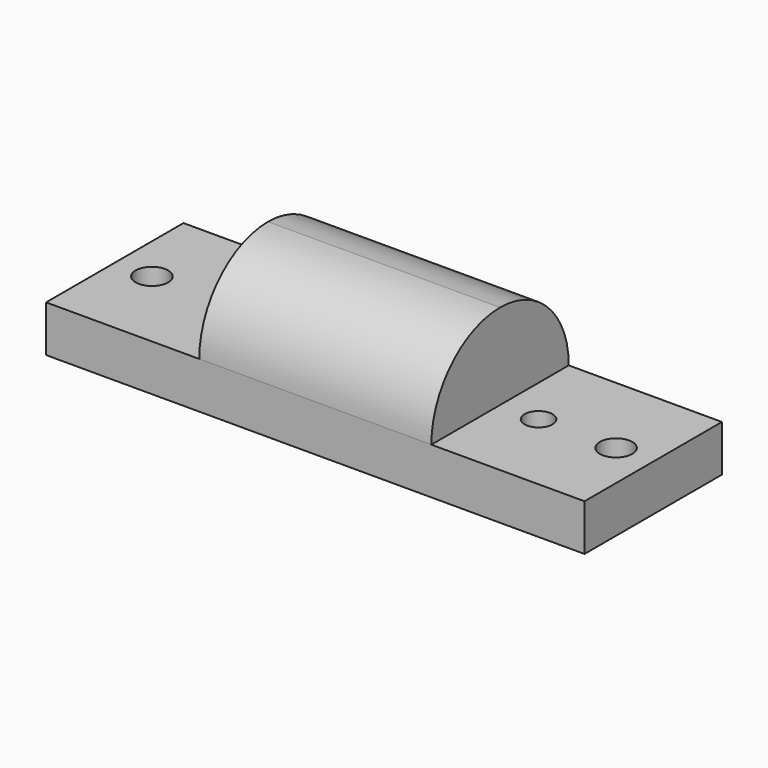
from build123d import *

# Parameters (mm, degrees)
F0_W     = 38
F0_H     = 18.5
F0_R     = 1.5
F0_W_2   = 10
F0_R_2   = 1.75
F1_DEPTH = 5
F2_W     = 25
F2_H     = 18.5
F3_DEPTH = 9.25
F5_DEPTH = 25


with BuildPart() as f1:
    # F0 (on Top) → F1 (new body)
    with BuildSketch(Plane.XY):
        Rectangle(F0_W, F0_H)
        with Locations((-16.65, 0)):
            Circle(F0_R, mode=Mode.SUBTRACT)
        with Locations((16.65, 0)):
            Circle(F0_R, mode=Mode.SUBTRACT)
        with Locations((24, 0)):
            Rectangle(F0_W_2, F0_H)
        with Locations((25, 0)):
            Circle(F0_R_2, mode=Mode.SUBTRACT)
        with Locations((-24, 0)):
            Rectangle(F0_W_2, F0_H)
        with Locations((-25, 0)):
            Circle(F0_R_2, mode=Mode.SUBTRACT)
    extrude(amount=F1_DEPTH)

    # F2 (on face) → F3 (join)
    with BuildSketch(Plane.XY.offset(5)):
        Rectangle(F2_W, F2_H)
    extrude(amount=F3_DEPTH)

    # F4 (on face) → F5 (cut)
    with BuildSketch(Plane(origin=(-12.5, 0, 0), x_dir=(0, -1, 0), z_dir=(-1, 0, 0))):
        with BuildLine():
            ThreePointArc((-9.25, 5), (-6.540737726, 11.540737726), (0, 14.25))
            Line((0, 14.25), (-9.25, 14.25))
            Line((-9.25, 14.25), (-9.25, 5))
        make_face()
        with BuildLine():
            ThreePointArc((0, 14.25), (6.540737726, 11.540737726), (9.25, 5))
            Line((9.25, 5), (9.25, 14.25))
            Line((9.25, 14.25), (0, 14.25))
        make_face()
    extrude(amount=-F5_DEPTH, mode=Mode.SUBTRACT)


solid = f1.part
